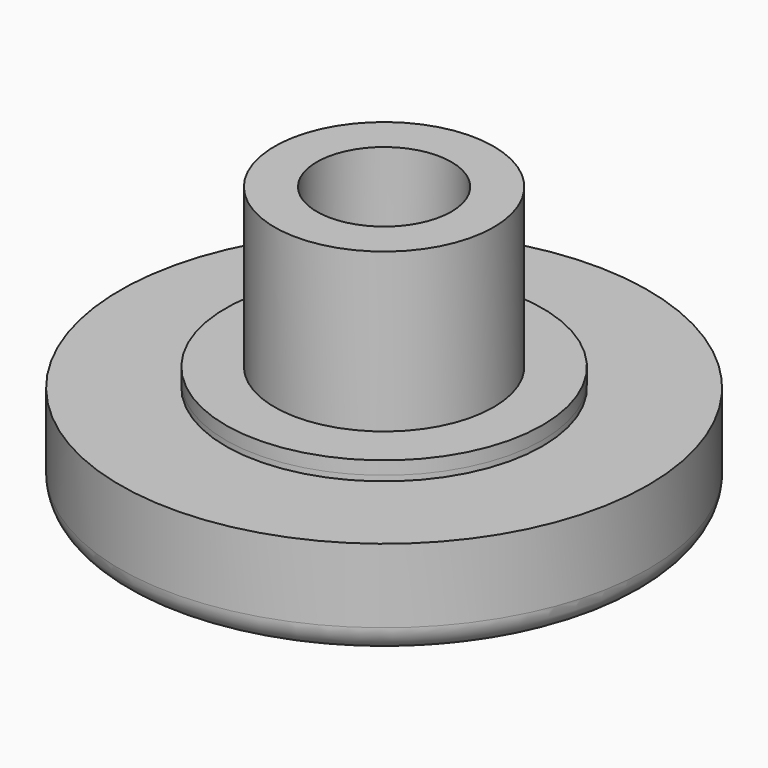
from build123d import *

# Parameters (mm, degrees)
F0_R     = 10
F0_R_2   = 6
F1_DEPTH = 4
F0_R_3   = 4.15
F0_R_4   = 2.55
F2_DEPTH = 10.5
F3_DEPTH = 4.5
F4_R     = 8.5
F4_R_2   = 6
F5_DEPTH = 1.5
F7_R     = 1
F8_DEPTH = 0.2


# Not quite as in the source:
# - a fillet or chamfer that OpenCascade refuses, or shapes differently, is made with other operations: its cross-section is extruded or revolved along the edge and cut away or added
# - a feature names something its author has since deleted; it is built from what else it names


with BuildPart() as f1:
    # F0 (on Top) → F1 (new body)
    with BuildSketch(Plane.XY):
        Circle(F0_R)
        Circle(F0_R_2, mode=Mode.SUBTRACT)
    extrude(amount=F1_DEPTH)



with BuildPart() as f1b:
    # F0 (on Top) → F1, piece 2 (new body)
    with BuildSketch(Plane.XY):
        Circle(F0_R_3)
        Circle(F0_R_4, mode=Mode.SUBTRACT)
        Circle(F0_R_4)
    extrude(amount=F1_DEPTH)

    # F0 (on Top) → F2 (join)
    with BuildSketch(Plane.XY):
        Circle(F0_R_3)
        Circle(F0_R_4, mode=Mode.SUBTRACT)
    extrude(amount=F2_DEPTH)


with BuildPart() as f1_1:
    add(f1.part)

    add(f1b.part)  # F3 merges F1b
    # F0 (on Top) → F3 (join)
    with BuildSketch(Plane.XY):
        Circle(F0_R_2)
        Circle(F0_R_3, mode=Mode.SUBTRACT)
    extrude(amount=F3_DEPTH)

    # F4 (on face) → F5 (cut)
    with BuildSketch(Plane.XY):
        Circle(F4_R)
        Circle(F4_R_2, mode=Mode.SUBTRACT)
        Circle(F4_R_2)
    extrude(amount=F5_DEPTH, mode=Mode.SUBTRACT)

    # F6: fillet of radius 20 on 1 edges, made by hand

    # F6_s1 → F6_t2 (revolve)
    with BuildSketch(Plane.XZ):
        with BuildLine():
            ThreePointArc((8.5, 0), (4.7736412694, 1.1214168703), (0.9006579232, 1.5))
            Line((0.9006579232, 1.5), (8.5, 1.5))
            Line((8.5, 1.5), (8.5, 0))
        make_face()
    revolve(axis=Axis((0, 0, 1.5), (0, 0, 1)))

    # F7
    f7_edges = [f1_1.edges().sort_by_distance(p)[0] for p in [
        (-10, 0, 0),
    ]]
    fillet(f7_edges, radius=F7_R)

    # F8 (cut): a face of the model
    f8_faces = [f1_1.faces().sort_by_distance(p)[0] for p in [
        (-9.7171572875, 0, 4),
    ]]
    extrude(f8_faces, amount=-F8_DEPTH, mode=Mode.SUBTRACT)


solid = f1_1.part
